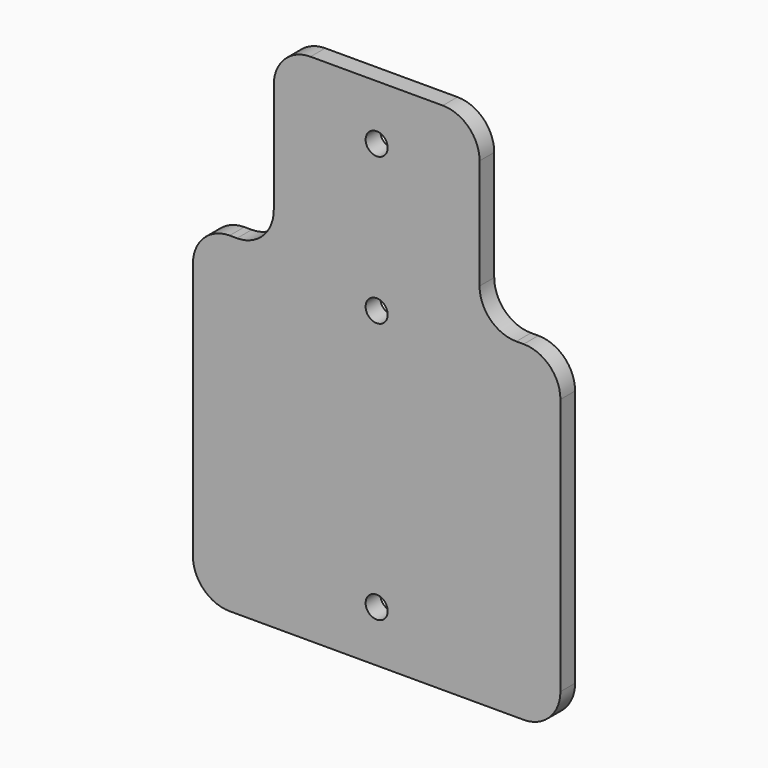
from build123d import *

# Parameters (mm, degrees)
F0_R     = 1.5
F1_DEPTH = 2.5
F2_R     = 5


with BuildPart() as f1:
    # F0 (on Front) → F1 (new body)
    with BuildSketch(Plane.XZ):
        Polygon((14, 10), (14, 35), (-14, 35), (-14, 10), (-25, 10), (-25, -35), (25, -35), (25, 10), align=None)
        with Locations((0, -28)):
            Circle(F0_R, mode=Mode.SUBTRACT)
        with Locations((0, 7.5)):
            Circle(F0_R, mode=Mode.SUBTRACT)
        with Locations((0, 27.5)):
            Circle(F0_R, mode=Mode.SUBTRACT)
    extrude(amount=F1_DEPTH)

    # F2
    f2_edges = [f1.edges().sort_by_distance(p)[0] for p in [
        (-14, -1.25, 10),
        (-25, -1.25, 10),
        (14, -1.25, 10),
        (25, -1.25, 10),
        (-25, -1.25, -35),
        (25, -1.25, -35),
        (14, -1.25, 35),
        (-14, -1.25, 35),
    ]]
    fillet(f2_edges, radius=F2_R)


solid = f1.part
